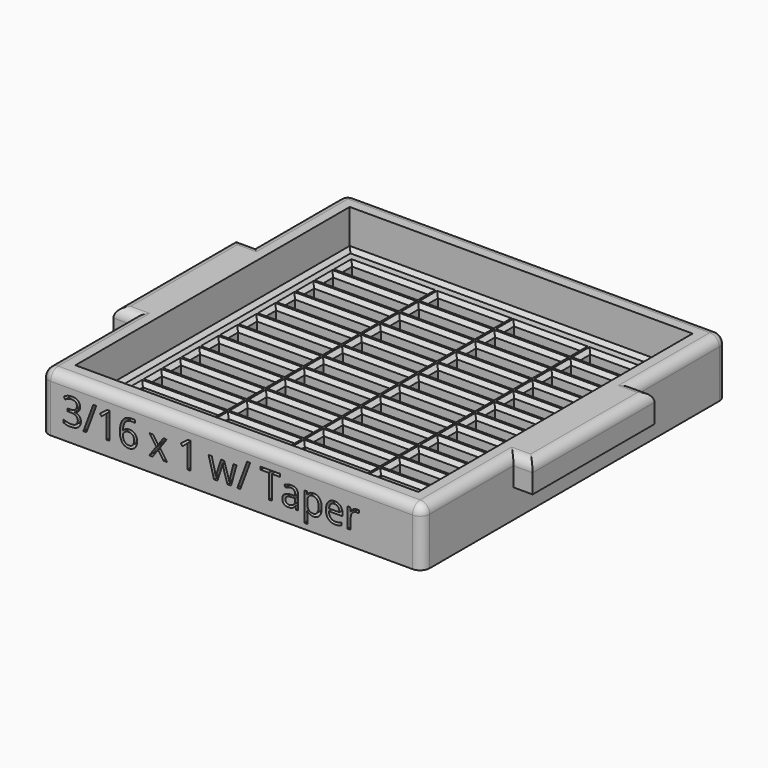
from build123d import *

# Parameters (mm, degrees)
F1_DEPTH     = 6.35
F0_W         = 6.35
F0_H         = 50.8
F2_DEPTH     = 19.05
F3_W         = 25.4
F3_H         = 4.7498
F3_W_2       = 22.225
F4_DEPTH     = 25.4
F5_R         = 3.175
F6_W         = 6.35
F6_H         = 50.8
F7_DEPTH     = 9.525
F8_SIZE      = 1.27
F9_TEXT_SIZE = 12.3223671431
F10_DEPTH    = 3.175


# Not quite as in the source:
# - a feature names something its author has since deleted; it is built from what else it names
# - Text() gives the source's letters only with a copy of the font that has no kerning and outlines rounded to 1/6400 em; it was checked with that copy


with BuildPart() as f1:
    # F0 (on Top) → F1 (new body)
    with BuildSketch(Plane.XY):
        Polygon((-57.15, 25.1415750563), (-57.15, -25.6584249437), (-57.15, -57.4084249437), (57.15, -57.4084249437), (57.15, -25.6584249437), (57.15, 25.1415750563), (57.15, 56.8915750563), (-57.15, 56.8915750563), align=None)
    extrude(amount=F1_DEPTH)

    # F0 (on Top) → F2 (join)
    with BuildSketch(Plane.XY):
        Polygon((-63.5, -25.6584249437), (-63.5, -63.7584249437), (63.5, -63.7584249437), (63.5, -25.6584249437), (57.15, -25.6584249437), (57.15, -57.4084249437), (-57.15, -57.4084249437), (-57.15, -25.6584249437), align=None)
        with Locations((-66.675, -0.2584249437)):
            Rectangle(F0_W, F0_H)
        with Locations((-60.325, -0.2584249437)):
            Rectangle(F0_W, F0_H)
        with Locations((60.325, -0.2584249437)):
            Rectangle(F0_W, F0_H)
        with Locations((66.675, -0.2584249437)):
            Rectangle(F0_W, F0_H)
        Polygon((-63.5, 63.2415750563), (-63.5, 25.1415750563), (-57.15, 25.1415750563), (-57.15, 56.8915750563), (57.15, 56.8915750563), (57.15, 25.1415750563), (63.5, 25.1415750563), (63.5, 63.2415750563), align=None)
    extrude(amount=F2_DEPTH)

    # F3 (on face) → F4 (cut)
    with BuildSketch(Plane.XY.offset(6.35)):
        with Locations((-39.7002, -45.5085249437)):
            Rectangle(F3_W, F3_H)
        with Locations((-39.7002, -37.5837249437)):
            Rectangle(F3_W, F3_H)
        with Locations((-39.7002, -29.6589249437)):
            Rectangle(F3_W, F3_H)
        with Locations((-39.7002, -21.7341249437)):
            Rectangle(F3_W, F3_H)
        with Locations((-39.7002, -13.8093249437)):
            Rectangle(F3_W, F3_H)
        with Locations((-39.7002, -5.8845249437)):
            Rectangle(F3_W, F3_H)
        with Locations((-39.7002, 2.0402750563)):
            Rectangle(F3_W, F3_H)
        with Locations((-39.7002, 9.9650750563)):
            Rectangle(F3_W, F3_H)
        with Locations((-39.7002, 17.8898750563)):
            Rectangle(F3_W, F3_H)
        with Locations((-39.7002, 25.8146750563)):
            Rectangle(F3_W, F3_H)
        with Locations((-39.7002, 33.7394750563)):
            Rectangle(F3_W, F3_H)
        with Locations((-39.7002, 41.6642750563)):
            Rectangle(F3_W, F3_H)
        with Locations((-39.7002, 49.5890750563)):
            Rectangle(F3_W, F3_H)
        with Locations((-12.7127, -45.5085249437)):
            Rectangle(F3_W_2, F3_H)
        with Locations((-12.7127, -37.5837249437)):
            Rectangle(F3_W_2, F3_H)
        with Locations((12.6873, -45.5085249437)):
            Rectangle(F3_W_2, F3_H)
        with Locations((12.6873, -37.5837249437)):
            Rectangle(F3_W_2, F3_H)
        with Locations((39.6748, -45.5085249437)):
            Rectangle(F3_W, F3_H)
        with Locations((39.6748, -37.5837249437)):
            Rectangle(F3_W, F3_H)
        with Locations((39.6748, -29.6589249437)):
            Rectangle(F3_W, F3_H)
        with Locations((39.6748, -21.7341249437)):
            Rectangle(F3_W, F3_H)
        with Locations((12.6873, -21.7341249437)):
            Rectangle(F3_W_2, F3_H)
        with Locations((12.6873, -29.6589249437)):
            Rectangle(F3_W_2, F3_H)
        with Locations((-12.7127, -29.6589249437)):
            Rectangle(F3_W_2, F3_H)
        with Locations((-12.7127, -21.7341249437)):
            Rectangle(F3_W_2, F3_H)
        with Locations((39.6748, -13.8093249437)):
            Rectangle(F3_W, F3_H)
        with Locations((39.6748, -5.8845249437)):
            Rectangle(F3_W, F3_H)
        with Locations((39.6748, 2.0402750563)):
            Rectangle(F3_W, F3_H)
        with Locations((12.6873, -13.8093249437)):
            Rectangle(F3_W_2, F3_H)
        with Locations((12.6873, -5.8845249437)):
            Rectangle(F3_W_2, F3_H)
        with Locations((12.6873, 2.0402750563)):
            Rectangle(F3_W_2, F3_H)
        with Locations((-12.7127, -13.8093249437)):
            Rectangle(F3_W_2, F3_H)
        with Locations((-12.7127, -5.8845249437)):
            Rectangle(F3_W_2, F3_H)
        with Locations((-12.7127, 2.0402750563)):
            Rectangle(F3_W_2, F3_H)
        with Locations((-12.7127, 9.9650750563)):
            Rectangle(F3_W_2, F3_H)
        with Locations((-12.7127, 17.8898750563)):
            Rectangle(F3_W_2, F3_H)
        with Locations((-12.7127, 25.8146750563)):
            Rectangle(F3_W_2, F3_H)
        with Locations((-12.7127, 33.7394750563)):
            Rectangle(F3_W_2, F3_H)
        with Locations((12.6873, 9.9650750563)):
            Rectangle(F3_W_2, F3_H)
        with Locations((12.6873, 17.8898750563)):
            Rectangle(F3_W_2, F3_H)
        with Locations((12.6873, 25.8146750563)):
            Rectangle(F3_W_2, F3_H)
        with Locations((12.6873, 33.7394750563)):
            Rectangle(F3_W_2, F3_H)
        with Locations((39.6748, 33.7394750563)):
            Rectangle(F3_W, F3_H)
        with Locations((39.6748, 25.8146750563)):
            Rectangle(F3_W, F3_H)
        with Locations((39.6748, 17.8898750563)):
            Rectangle(F3_W, F3_H)
        with Locations((39.6748, 9.9650750563)):
            Rectangle(F3_W, F3_H)
        with Locations((-12.7127, 41.6642750563)):
            Rectangle(F3_W_2, F3_H)
        with Locations((-12.7127, 49.5890750563)):
            Rectangle(F3_W_2, F3_H)
        with Locations((12.6873, 49.5890750563)):
            Rectangle(F3_W_2, F3_H)
        with Locations((12.6873, 41.6642750563)):
            Rectangle(F3_W_2, F3_H)
        with Locations((39.6748, 41.6642750563)):
            Rectangle(F3_W, F3_H)
        with Locations((39.6748, 49.5890750563)):
            Rectangle(F3_W, F3_H)
    extrude(amount=-F4_DEPTH, mode=Mode.SUBTRACT)

    # F5
    f5_edges = [f1.edges().sort_by_distance(p)[0] for p in [
        (-63.5, -44.708425, 19.05),
        (0, -63.758425, 19.05),
        (63.5, -44.708425, 19.05),
        (66.675, -25.658425, 19.05),
        (69.85, -0.258425, 19.05),
        (-66.675, -25.658425, 19.05),
        (-69.85, -0.258425, 19.05),
        (-66.675, 25.141575, 19.05),
        (-63.5, 44.191575, 19.05),
        (0, 63.241575, 19.05),
        (63.5, 44.191575, 19.05),
        (66.675, 25.141575, 19.05),
        (63.5, -63.758425, 9.525),
        (-63.5, -63.758425, 9.525),
        (-63.5, 63.241575, 9.525),
        (63.5, 63.241575, 9.525),
    ]]
    fillet(f5_edges, radius=F5_R)

    # F6 (on face) → F7 (cut)
    with BuildSketch(Plane(origin=(0, 0, 0), x_dir=(1, 0, 0), z_dir=(0, 0, -1))):
        with Locations((-66.675, 0.2584249437)):
            Rectangle(F6_W, F6_H)
        with Locations((66.675, 0.2584249437)):
            Rectangle(F6_W, F6_H)
    extrude(amount=-F7_DEPTH, mode=Mode.SUBTRACT)

    # F8
    f8_edges = [f1.edges().sort_by_distance(p)[0] for p in [
        (-57.15, -0.258425, 6.35),
        (0, -57.408425, 6.35),
        (0, 56.891575, 6.35),
        (57.15, -0.258425, 6.35),
        (-52.4002, -45.508525, 6.35),
        (-39.7002, -47.883425, 6.35),
        (-27.0002, -45.508525, 6.35),
        (-39.7002, -43.133625, 6.35),
        (-52.4002, -37.583725, 6.35),
        (-39.7002, -39.958625, 6.35),
        (-27.0002, -37.583725, 6.35),
        (-39.7002, -35.208825, 6.35),
        (-52.4002, -29.658925, 6.35),
        (-39.7002, -32.033825, 6.35),
        (-27.0002, -29.658925, 6.35),
        (-39.7002, -27.284025, 6.35),
        (-12.7127, -43.133625, 6.35),
        (-23.8252, -45.508525, 6.35),
        (-12.7127, -47.883425, 6.35),
        (-1.6002, -45.508525, 6.35),
        (-12.7127, -35.208825, 6.35),
        (-23.8252, -37.583725, 6.35),
        (-12.7127, -39.958625, 6.35),
        (-1.6002, -37.583725, 6.35),
        (-12.7127, -27.284025, 6.35),
        (-23.8252, -29.658925, 6.35),
        (-12.7127, -32.033825, 6.35),
        (-1.6002, -29.658925, 6.35),
        (-52.4002, -21.734125, 6.35),
        (-39.7002, -24.109025, 6.35),
        (-27.0002, -21.734125, 6.35),
        (-39.7002, -19.359225, 6.35),
        (-52.4002, -13.809325, 6.35),
        (-39.7002, -16.184225, 6.35),
        (-27.0002, -13.809325, 6.35),
        (-39.7002, -11.434425, 6.35),
        (-52.4002, -5.884525, 6.35),
        (-39.7002, -8.259425, 6.35),
        (-27.0002, -5.884525, 6.35),
        (-39.7002, -3.509625, 6.35),
        (-52.4002, 2.040275, 6.35),
        (-39.7002, -0.334625, 6.35),
        (-27.0002, 2.040275, 6.35),
        (-39.7002, 4.415175, 6.35),
        (-12.7127, -19.359225, 6.35),
        (-23.8252, -21.734125, 6.35),
        (-12.7127, -24.109025, 6.35),
        (-1.6002, -21.734125, 6.35),
        (-12.7127, -11.434425, 6.35),
        (-23.8252, -13.809325, 6.35),
        (-12.7127, -16.184225, 6.35),
        (-1.6002, -13.809325, 6.35),
        (-12.7127, -3.509625, 6.35),
        (-23.8252, -5.884525, 6.35),
        (-12.7127, -8.259425, 6.35),
        (-1.6002, -5.884525, 6.35),
        (1.5748, -45.508525, 6.35),
        (12.6873, -47.883425, 6.35),
        (23.7998, -45.508525, 6.35),
        (12.6873, -43.133625, 6.35),
        (1.5748, -37.583725, 6.35),
        (12.6873, -39.958625, 6.35),
        (23.7998, -37.583725, 6.35),
        (12.6873, -35.208825, 6.35),
        (1.5748, -29.658925, 6.35),
        (12.6873, -32.033825, 6.35),
        (23.7998, -29.658925, 6.35),
        (12.6873, -27.284025, 6.35),
        (26.9748, -45.508525, 6.35),
        (39.6748, -47.883425, 6.35),
        (52.3748, -45.508525, 6.35),
        (39.6748, -43.133625, 6.35),
        (26.9748, -37.583725, 6.35),
        (39.6748, -39.958625, 6.35),
        (52.3748, -37.583725, 6.35),
        (39.6748, -35.208825, 6.35),
        (26.9748, -29.658925, 6.35),
        (39.6748, -32.033825, 6.35),
        (52.3748, -29.658925, 6.35),
        (39.6748, -27.284025, 6.35),
        (1.5748, -21.734125, 6.35),
        (12.6873, -24.109025, 6.35),
        (23.7998, -21.734125, 6.35),
        (12.6873, -19.359225, 6.35),
        (1.5748, -13.809325, 6.35),
        (12.6873, -16.184225, 6.35),
        (23.7998, -13.809325, 6.35),
        (12.6873, -11.434425, 6.35),
        (1.5748, -5.884525, 6.35),
        (12.6873, -8.259425, 6.35),
        (23.7998, -5.884525, 6.35),
        (12.6873, -3.509625, 6.35),
        (26.9748, -21.734125, 6.35),
        (39.6748, -24.109025, 6.35),
        (52.3748, -21.734125, 6.35),
        (39.6748, -19.359225, 6.35),
        (26.9748, -13.809325, 6.35),
        (39.6748, -16.184225, 6.35),
        (52.3748, -13.809325, 6.35),
        (39.6748, -11.434425, 6.35),
        (26.9748, -5.884525, 6.35),
        (39.6748, -8.259425, 6.35),
        (52.3748, -5.884525, 6.35),
        (39.6748, -3.509625, 6.35),
        (-52.4002, 9.965075, 6.35),
        (-39.7002, 7.590175, 6.35),
        (-27.0002, 9.965075, 6.35),
        (-39.7002, 12.339975, 6.35),
        (-52.4002, 17.889875, 6.35),
        (-39.7002, 15.514975, 6.35),
        (-27.0002, 17.889875, 6.35),
        (-39.7002, 20.264775, 6.35),
        (-52.4002, 25.814675, 6.35),
        (-39.7002, 23.439775, 6.35),
        (-27.0002, 25.814675, 6.35),
        (-39.7002, 28.189575, 6.35),
        (-12.7127, 4.415175, 6.35),
        (-23.8252, 2.040275, 6.35),
        (-12.7127, -0.334625, 6.35),
        (-1.6002, 2.040275, 6.35),
        (-12.7127, 12.339975, 6.35),
        (-23.8252, 9.965075, 6.35),
        (-12.7127, 7.590175, 6.35),
        (-1.6002, 9.965075, 6.35),
        (-12.7127, 20.264775, 6.35),
        (-23.8252, 17.889875, 6.35),
        (-12.7127, 15.514975, 6.35),
        (-1.6002, 17.889875, 6.35),
        (-12.7127, 28.189575, 6.35),
        (-23.8252, 25.814675, 6.35),
        (-12.7127, 23.439775, 6.35),
        (-1.6002, 25.814675, 6.35),
        (-52.4002, 33.739475, 6.35),
        (-39.7002, 31.364575, 6.35),
        (-27.0002, 33.739475, 6.35),
        (-39.7002, 36.114375, 6.35),
        (-52.4002, 41.664275, 6.35),
        (-39.7002, 39.289375, 6.35),
        (-27.0002, 41.664275, 6.35),
        (-39.7002, 44.039175, 6.35),
        (-52.4002, 49.589075, 6.35),
        (-39.7002, 47.214175, 6.35),
        (-27.0002, 49.589075, 6.35),
        (-39.7002, 51.963975, 6.35),
        (-12.7127, 36.114375, 6.35),
        (-23.8252, 33.739475, 6.35),
        (-12.7127, 31.364575, 6.35),
        (-1.6002, 33.739475, 6.35),
        (-12.7127, 44.039175, 6.35),
        (-23.8252, 41.664275, 6.35),
        (-12.7127, 39.289375, 6.35),
        (-1.6002, 41.664275, 6.35),
        (-12.7127, 51.963975, 6.35),
        (-23.8252, 49.589075, 6.35),
        (-12.7127, 47.214175, 6.35),
        (-1.6002, 49.589075, 6.35),
        (1.5748, 2.040275, 6.35),
        (12.6873, -0.334625, 6.35),
        (23.7998, 2.040275, 6.35),
        (12.6873, 4.415175, 6.35),
        (1.5748, 9.965075, 6.35),
        (12.6873, 7.590175, 6.35),
        (23.7998, 9.965075, 6.35),
        (12.6873, 12.339975, 6.35),
        (1.5748, 17.889875, 6.35),
        (12.6873, 15.514975, 6.35),
        (23.7998, 17.889875, 6.35),
        (12.6873, 20.264775, 6.35),
        (1.5748, 25.814675, 6.35),
        (12.6873, 23.439775, 6.35),
        (23.7998, 25.814675, 6.35),
        (12.6873, 28.189575, 6.35),
        (26.9748, 2.040275, 6.35),
        (39.6748, -0.334625, 6.35),
        (52.3748, 2.040275, 6.35),
        (39.6748, 4.415175, 6.35),
        (26.9748, 9.965075, 6.35),
        (39.6748, 7.590175, 6.35),
        (52.3748, 9.965075, 6.35),
        (39.6748, 12.339975, 6.35),
        (26.9748, 17.889875, 6.35),
        (39.6748, 15.514975, 6.35),
        (52.3748, 17.889875, 6.35),
        (39.6748, 20.264775, 6.35),
        (26.9748, 25.814675, 6.35),
        (39.6748, 23.439775, 6.35),
        (52.3748, 25.814675, 6.35),
        (39.6748, 28.189575, 6.35),
        (1.5748, 33.739475, 6.35),
        (12.6873, 31.364575, 6.35),
        (23.7998, 33.739475, 6.35),
        (12.6873, 36.114375, 6.35),
        (1.5748, 41.664275, 6.35),
        (12.6873, 39.289375, 6.35),
        (23.7998, 41.664275, 6.35),
        (12.6873, 44.039175, 6.35),
        (1.5748, 49.589075, 6.35),
        (12.6873, 47.214175, 6.35),
        (23.7998, 49.589075, 6.35),
        (12.6873, 51.963975, 6.35),
        (26.9748, 33.739475, 6.35),
        (39.6748, 31.364575, 6.35),
        (52.3748, 33.739475, 6.35),
        (39.6748, 36.114375, 6.35),
        (26.9748, 41.664275, 6.35),
        (39.6748, 39.289375, 6.35),
        (52.3748, 41.664275, 6.35),
        (39.6748, 44.039175, 6.35),
        (26.9748, 49.589075, 6.35),
        (39.6748, 47.214175, 6.35),
        (52.3748, 49.589075, 6.35),
        (39.6748, 51.963975, 6.35),
    ]]
    chamfer(f8_edges, length=F8_SIZE)

    # F9 (on face) → F10 (cut)
    with BuildSketch(Plane.XZ.offset(63.7584249437)):
        with Locations((-56.5712153912, 4.8063991126)):
            Text('3/16 x 1 w/ Taper', F9_TEXT_SIZE, font='Open Sans', text_align=(TextAlign.LEFT, TextAlign.BOTTOM))
    extrude(amount=-F10_DEPTH, mode=Mode.SUBTRACT)


solid = f1.part
